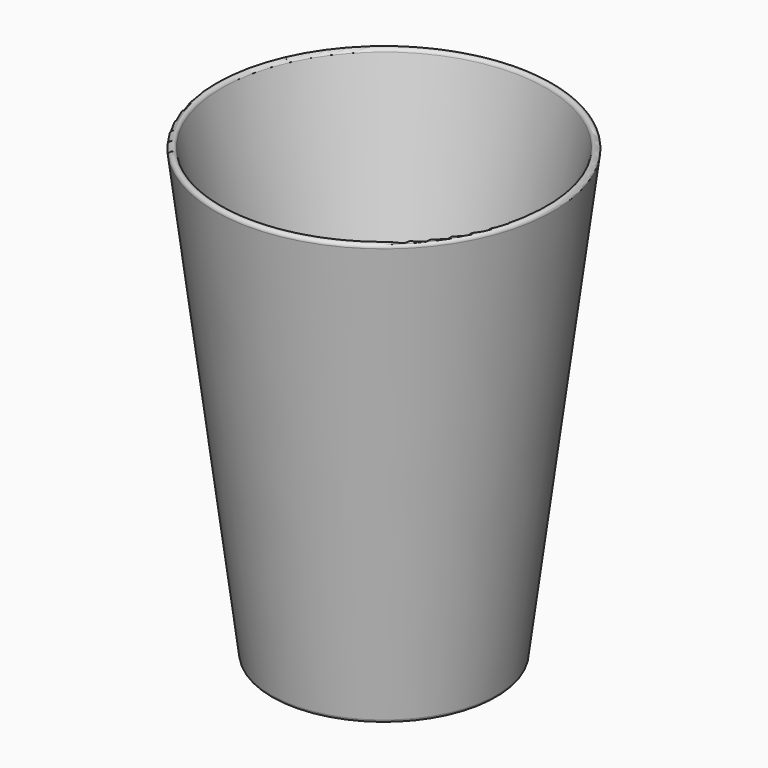
from build123d import *

# Parameters (mm, degrees)
F3_R = 1.5875


# Not quite as in the source:
# - a variable given as a bare number and used for a length is read in inches; the dataset says mm whatever the document's units were


with BuildPart() as f2:
    # F1 (on Front) → F2 (revolve)
    with BuildSketch(Plane.XZ):
        with BuildLine():
            Line((-50.8, 0), (0, 0))
            Line((0, 0), (0, 3.175))
            Line((0, 3.175), (-29.0172447749, 3.175))
            Line((-29.0172447749, 3.175), (-73.0551675175, 201.8488507874))
            ThreePointArc((-73.0551675175, 201.8488507874), (-74.8424777646, 203.1850293835), (-76.2, 201.4138759344))
            Line((-76.2, 201.4138759344), (-50.8, 0))
        make_face()
    revolve(axis=Axis((0, 0, 1.5875), (0, 0, -1)))

    # F3
    f3_edges = [f2.edges().sort_by_distance(p)[0] for p in [
        (50.8, 0, 0),
        (29.017245, 0, 3.175),
    ]]
    fillet(f3_edges, radius=F3_R)


solid = f2.part
